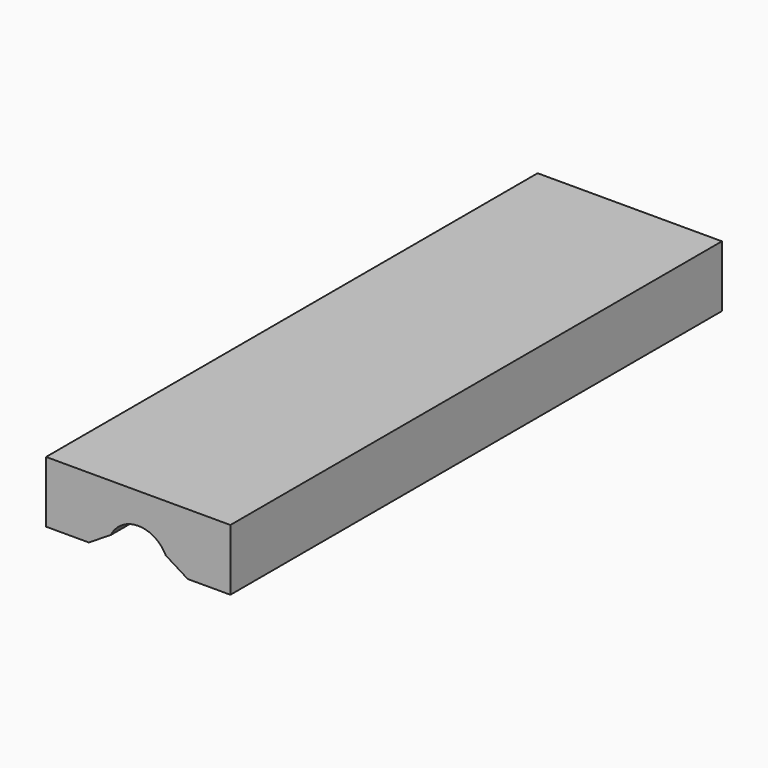
from build123d import *

# Parameters (mm, degrees)
F1_DEPTH    = 50
F2_T1_DEPTH = 57.9983578358


# Not quite as in the source:
# - a fillet or chamfer that OpenCascade refuses, or shapes differently, is made with other operations: its cross-section is extruded or revolved along the edge and cut away or added


with BuildPart() as f1:
    # F0 (on Front) → F1 (new body)
    with BuildSketch(Plane.XZ):
        with BuildLine():
            Line((7.5, 5), (0, 5))
            Line((0, 5), (-7.5, 5))
            Line((-7.5, 5), (-7.5, 0))
            Line((-7.5, 0), (-2.5, 0))
            ThreePointArc((-2.5, 0), (-1.767766953, 1.767766953), (0, 2.5))
            ThreePointArc((0, 2.5), (1.767766953, 1.767766953), (2.5, 0))
            Line((2.5, 0), (7.5, 0))
            Line((7.5, 0), (7.5, 5))
        make_face()
    extrude(amount=F1_DEPTH)

    # F2: chamfer of 2 on 2 edges, made by hand

    # F2_s2 → F2_t1 (cut)
    with BuildSketch(Plane.XZ.offset(-3.9991789179)):
        with BuildLine():
            Line((-4.0311288741, 0), (-2.2395160412, 1.1111111111))
            ThreePointArc((-2.2395160412, 1.1111111111), (-2.4271314798, 0.5991934409), (-2.5, 0))
            Line((-2.5, 0), (-4.0311288741, 0))
        make_face()
        with BuildLine():
            Line((4.0311288741, 0), (2.2395160412, 1.1111111111))
            ThreePointArc((2.2395160412, 1.1111111111), (2.4271314798, 0.5991934409), (2.5, 0))
            Line((2.5, 0), (4.0311288741, 0))
        make_face()
    extrude(amount=F2_T1_DEPTH, mode=Mode.SUBTRACT)


solid = f1.part
